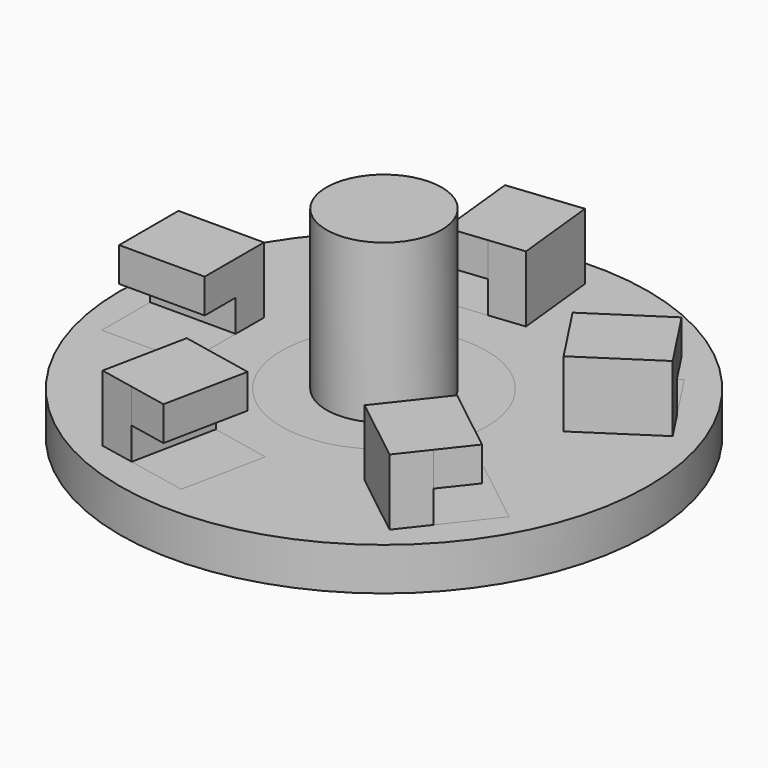
from build123d import *

# Parameters (mm, degrees)
F0_R      = 23.155
F0_R_2    = 9
F1_DEPTH  = 3.75
F0_R_3    = 6.3
F2_DEPTH  = 4.75
F3_DEPTH  = 5.8
F4_DEPTH  = 3.75
F5_W      = 7.5
F5_H      = 3
F6_DEPTH  = 3.4
F0_W      = 7.5
F0_H      = 3.1
F7_DEPTH  = 5.8
F8_W      = 7.5
F8_H      = 3
F9_DEPTH  = 3.4
F10_W     = 7.5
F10_H     = 3
F11_DEPTH = 3.4
F12_DEPTH = 3.75
F13_W     = 7.5
F13_H     = 3
F14_DEPTH = 3.4
F15_W     = 7.5
F15_H     = 3
F16_DEPTH = 3.4
F0_R_4    = 5.05
F17_DEPTH = 3.75
F18_DEPTH = 3.75
F19_DEPTH = 11.9
F20_R     = 5.05
F21_DEPTH = 2
F22_DEPTH = 3.75
F0_H_2    = 5.3


with BuildPart() as f1:
    # F0 (on Top) → F1 (new body)
    with BuildSketch(Plane.XY):
        Circle(F0_R)
        Polygon((-8.2636521274, -11.2850000563), (-5.2259463077, -11.9033392453), (-0.032449261, -12.9604997943), (-1.5284311699, -20.3097880678), (-6.7219282165, -19.2526275189), (-9.7596340363, -18.6342883299), align=None, mode=Mode.SUBTRACT)
        Polygon((-13, 3.1), (-13, 0), (-13, -5.3), (-20.5, -5.3), (-20.5, 0), (-20.5, 3.1), align=None, mode=Mode.SUBTRACT)
        Polygon((7.4554983603, -11.4469093574), (9.3713907755, -9.0098299058), (12.6469487758, -4.8432101983), (18.5431087392, -9.4784337836), (15.267550739, -13.6450534911), (13.3516583238, -16.0821329427), align=None, mode=Mode.SUBTRACT)
        Polygon((1.8337635187, 13.2682430609), (-1.2487967823, 12.9398804707), (-4.8285442287, 12.5585561724), (-6.5189805228, 12.3784863649), (-7.3134061442, 19.8362935448), (-5.6229698501, 20.0163633523), (-2.0432224037, 20.3976876506), (1.0393378973, 20.7260502408), align=None, mode=Mode.SUBTRACT)
        Circle(F0_R_2, mode=Mode.SUBTRACT)
        Polygon((13.5594344097, 2.734427086), (11.8587776603, 5.3262925571), (8.9512032177, 9.7575464271), (15.2218454866, 13.8720385629), (18.1294199292, 9.4407846929), (19.8300766787, 6.8489192217), align=None, mode=Mode.SUBTRACT)
    extrude(amount=-F1_DEPTH)

    # F0 (on Top) → F4 (join)
    with BuildSketch(Plane.XY):
        Polygon((-2.0432224037, 20.3976876506), (-1.2487967823, 12.9398804707), (1.8337635187, 13.2682430609), (1.0393378973, 20.7260502408), align=None)
    extrude(amount=-F4_DEPTH)


with BuildPart() as f2:
    # F0 (on Top) → F2 (new body)
    with BuildSketch(Plane.XY):
        Circle(F0_R_2)
        Circle(F0_R_3, mode=Mode.SUBTRACT)
    extrude(amount=-F2_DEPTH)

    # F0 (on Top) → F17 (join)
    with BuildSketch(Plane.XY):
        Circle(F0_R_3)
        Circle(F0_R_4, mode=Mode.SUBTRACT)
    extrude(amount=-F17_DEPTH)

    # F0 (on Top) → F18 (join)
    with BuildSketch(Plane.XY):
        Circle(F0_R_4)
        with BuildLine():
            Line((2.7389110228, 2.575), (2.7389110228, -2.575))
            ThreePointArc((2.7389110228, -2.575), (1.491993259, -3.4505383211), (0, -3.7592896391))
            ThreePointArc((0, -3.7592896391), (-1.491993259, -3.4505383211), (-2.7389110228, -2.575))
            Line((-2.7389110228, -2.575), (-2.7389110228, 2.575))
            ThreePointArc((-2.7389110228, 2.575), (-1.491993259, 3.4505383211), (0, 3.7592896391))
            ThreePointArc((0, 3.7592896391), (1.491993259, 3.4505383211), (2.7389110228, 2.575))
        make_face(mode=Mode.SUBTRACT)
    extrude(amount=-F18_DEPTH)

    # F0 (on Top) → F19 (join)
    with BuildSketch(Plane.XY):
        Circle(F0_R_4)
        with BuildLine():
            Line((2.7389110228, 2.575), (2.7389110228, -2.575))
            ThreePointArc((2.7389110228, -2.575), (1.491993259, -3.4505383211), (0, -3.7592896391))
            ThreePointArc((0, -3.7592896391), (-1.491993259, -3.4505383211), (-2.7389110228, -2.575))
            Line((-2.7389110228, -2.575), (-2.7389110228, 2.575))
            ThreePointArc((-2.7389110228, 2.575), (-1.491993259, 3.4505383211), (0, 3.7592896391))
            ThreePointArc((0, 3.7592896391), (1.491993259, 3.4505383211), (2.7389110228, 2.575))
        make_face(mode=Mode.SUBTRACT)
    extrude(amount=F19_DEPTH)

    # F20 (on face) → F21 (join)
    with BuildSketch(Plane.XY.offset(11.9)):
        Circle(F20_R)
        with BuildLine():
            Line((-2.7389110228, -2.575), (-2.7389110228, 2.575))
            ThreePointArc((-2.7389110228, 2.575), (0, 3.7592896391), (2.7389110228, 2.575))
            Line((2.7389110228, 2.575), (2.7389110228, -2.575))
            ThreePointArc((2.7389110228, -2.575), (0, -3.7592896391), (-2.7389110228, -2.575))
        make_face(mode=Mode.SUBTRACT)
        with BuildLine():
            ThreePointArc((2.7389110228, 2.575), (0, 3.7592896391), (-2.7389110228, 2.575))
            Line((-2.7389110228, 2.575), (-2.7389110228, -2.575))
            ThreePointArc((-2.7389110228, -2.575), (0, -3.7592896391), (2.7389110228, -2.575))
            Line((2.7389110228, -2.575), (2.7389110228, 2.575))
        make_face()
    extrude(amount=F21_DEPTH)


with BuildPart() as f3:
    # F0 (on Top) → F3 (new body)
    with BuildSketch(Plane.XY):
        Polygon((-2.0432224037, 20.3976876506), (-1.2487967823, 12.9398804707), (1.8337635187, 13.2682430609), (1.0393378973, 20.7260502408), align=None)
    extrude(amount=F3_DEPTH)

    # F5 (on face) → F6 (join)
    with BuildSketch(Plane(origin=(0.1281399733, 0.0136498136, 0), x_dir=(0.1059234162, -0.9943742906, 0), z_dir=(-0.9943742906, -0.1059234162, 0))):
        with Locations((-16.7493612855, 4.3)):
            Rectangle(F5_W, F5_H)
    extrude(amount=F6_DEPTH)


with BuildPart() as f7:
    # F0 (on Top) → F7 (new body)
    with BuildSketch(Plane.XY):
        with Locations((-16.75, 1.55)):
            Rectangle(F0_W, F0_H)
    extrude(amount=F7_DEPTH)

    # F8 (on face) → F9 (join)
    with BuildSketch(Plane.XZ):
        with Locations((-16.75, 4.3)):
            Rectangle(F8_W, F8_H)
    extrude(amount=F9_DEPTH)


with BuildPart() as f7b:
    # F0 (on Top) → F7, piece 2 (new body)
    with BuildSketch(Plane.XY):
        Polygon((18.1294199292, 9.4407846929), (11.8587776603, 5.3262925571), (13.5594344097, 2.734427086), (19.8300766787, 6.8489192217), align=None)
    extrude(amount=F7_DEPTH)

    # F15 (on face) → F16 (join)
    with BuildSketch(Plane(origin=(1.1259863408, -1.7160459443, 0), x_dir=(-0.8360856359, -0.5485989514, 0), z_dir=(-0.5485989514, 0.8360856359, 0))):
        with Locations((-16.5869521724, 4.3)):
            Rectangle(F15_W, F15_H)
    extrude(amount=F16_DEPTH)


with BuildPart() as f7c:
    # F0 (on Top) → F7, piece 3 (new body)
    with BuildSketch(Plane.XY):
        Polygon((15.267550739, -13.6450534911), (9.3713907755, -9.0098299058), (7.4554983603, -11.4469093574), (13.3516583238, -16.0821329427), align=None)
    extrude(amount=F7_DEPTH)

    # F13 (on face) → F14 (join)
    with BuildSketch(Plane(origin=(-0.7980748179, -1.0151779526, 0), x_dir=(-0.7861546618, 0.6180298114, 0), z_dir=(0.6180298114, 0.7861546618, 0))):
        with Locations((-16.6857060228, 4.3)):
            Rectangle(F13_W, F13_H)
    extrude(amount=F14_DEPTH)


with BuildPart() as f7d:
    # F0 (on Top) → F7, piece 4 (new body)
    with BuildSketch(Plane.XY):
        Polygon((-6.7219282165, -19.2526275189), (-5.2259463077, -11.9033392453), (-8.2636521274, -11.2850000563), (-9.7596340363, -18.6342883299), align=None)
    extrude(amount=F7_DEPTH)

    # F10 (on face) → F11 (join)
    with BuildSketch(Plane(origin=(-2.6914473039, 0.547856653, 0), x_dir=(0.1994642545, 0.9799051031, 0), z_dir=(0.9799051031, -0.1994642545, 0))):
        with Locations((-16.4565323554, 4.3)):
            Rectangle(F10_W, F10_H)
    extrude(amount=F11_DEPTH)


with BuildPart() as f12:
    # F0 (on Top) → F12 (new body)
    with BuildSketch(Plane.XY):
        with Locations((-16.75, 1.55)):
            Rectangle(F0_W, F0_H)
    extrude(amount=-F12_DEPTH)


with BuildPart() as f12b:
    # F0 (on Top) → F12, piece 2 (new body)
    with BuildSketch(Plane.XY):
        Polygon((-6.7219282165, -19.2526275189), (-5.2259463077, -11.9033392453), (-8.2636521274, -11.2850000563), (-9.7596340363, -18.6342883299), align=None)
    extrude(amount=-F12_DEPTH)


with BuildPart() as f12c:
    # F0 (on Top) → F12, piece 3 (new body)
    with BuildSketch(Plane.XY):
        Polygon((18.1294199292, 9.4407846929), (11.8587776603, 5.3262925571), (13.5594344097, 2.734427086), (19.8300766787, 6.8489192217), align=None)
    extrude(amount=-F12_DEPTH)


with BuildPart() as f12d:
    # F0 (on Top) → F12, piece 4 (new body)
    with BuildSketch(Plane.XY):
        Polygon((15.267550739, -13.6450534911), (9.3713907755, -9.0098299058), (7.4554983603, -11.4469093574), (13.3516583238, -16.0821329427), align=None)
    extrude(amount=-F12_DEPTH)


with BuildPart() as f22:
    # F0 (on Top) → F22 (new body)
    with BuildSketch(Plane.XY):
        Polygon((-6.5189805228, 12.3784863649), (-4.8285442287, 12.5585561724), (-5.6229698501, 20.0163633523), (-7.3134061442, 19.8362935448), align=None)
        Polygon((-4.8285442287, 12.5585561724), (-1.2487967823, 12.9398804707), (-2.0432224037, 20.3976876506), (-5.6229698501, 20.0163633523), align=None)
    extrude(amount=-F22_DEPTH)


with BuildPart() as f22b:
    # F0 (on Top) → F22, piece 2 (new body)
    with BuildSketch(Plane.XY):
        with Locations((-16.75, -2.65)):
            Rectangle(F0_W, F0_H_2)
    extrude(amount=-F22_DEPTH)


with BuildPart() as f22c:
    # F0 (on Top) → F22, piece 3 (new body)
    with BuildSketch(Plane.XY):
        Polygon((-0.032449261, -12.9604997943), (-5.2259463077, -11.9033392453), (-6.7219282165, -19.2526275189), (-1.5284311699, -20.3097880678), align=None)
    extrude(amount=-F22_DEPTH)


with BuildPart() as f22d:
    # F0 (on Top) → F22, piece 4 (new body)
    with BuildSketch(Plane.XY):
        Polygon((12.6469487758, -4.8432101983), (9.3713907755, -9.0098299058), (15.267550739, -13.6450534911), (18.5431087392, -9.4784337836), align=None)
    extrude(amount=-F22_DEPTH)


with BuildPart() as f22e:
    # F0 (on Top) → F22, piece 5 (new body)
    with BuildSketch(Plane.XY):
        Polygon((8.9512032177, 9.7575464271), (11.8587776603, 5.3262925571), (18.1294199292, 9.4407846929), (15.2218454866, 13.8720385629), align=None)
    extrude(amount=-F22_DEPTH)


solid = Compound([f1.part, f2.part, f3.part, f7.part, f7b.part, f7c.part, f7d.part, f12.part, f12b.part, f12c.part, f12d.part, f22.part, f22b.part, f22c.part, f22d.part, f22e.part])
